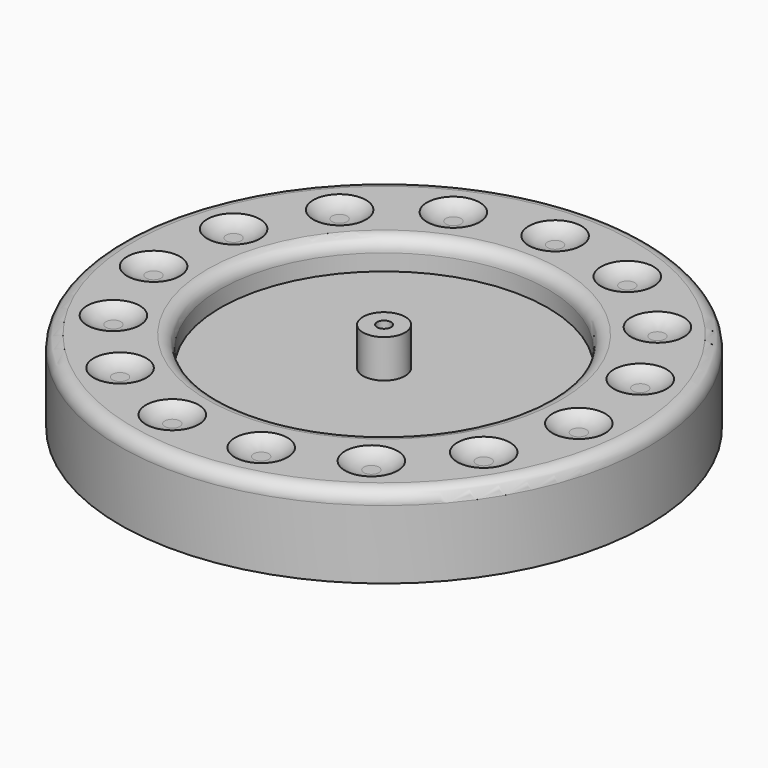
from build123d import *

# Parameters (mm, degrees)
F0_R      = 50
F1_DEPTH  = 15.5
F2_R      = 31
F3_DEPTH  = 7.1
F4_R      = 11.125
F5_DEPTH  = 9
F6_R      = 2.5
F7_R      = 5
F8_DEPTH  = 1.5
F10_R     = 31.0625
F11_DEPTH = 1.5
F12_R     = 4
F13_DEPTH = 7.25
F15_D     = 2.65
F15_DEPTH = 10
F15_TIP   = 0.7961403202


# Not quite as in the source:
# - a fillet or chamfer that OpenCascade refuses, or shapes differently, is made with other operations: its cross-section is extruded or revolved along the edge and cut away or added


with BuildPart() as f1:
    # F0 (on Top) → F1 (new body)
    with BuildSketch(Plane.XY):
        Circle(F0_R)
    extrude(amount=F1_DEPTH)

    # F2 (on face) → F3 (cut)
    with BuildSketch(Plane.XY.offset(15.5)):
        Circle(F2_R)
    extrude(amount=-F3_DEPTH, mode=Mode.SUBTRACT)

    # F4 (on face) → F5 (cut)
    with BuildSketch(Plane.XY.offset(8.4)):
        Circle(F4_R)
    extrude(amount=-F5_DEPTH, mode=Mode.SUBTRACT)

    # F6
    f6_edges = [f1.edges().sort_by_distance(p)[0] for p in [
        (-50, 0, 15.5),
        (-31, 0, 15.5),
    ]]
    fillet(f6_edges, radius=F6_R)

    # F7 (on face) → F8 (cut)
    with BuildSketch(Plane.XY.offset(15.5)):
        with Locations((0, 40.5)):
            Circle(F7_R)
        with Locations((-16.4728340446, 36.9985910345)):
            Circle(F7_R)
        with Locations((-30.0973654318, 27.0997895575)):
            Circle(F7_R)
        with Locations((-38.51778891, 12.5151882722)):
            Circle(F7_R)
        with Locations((-40.2781367624, -4.2334027623)):
            Circle(F7_R)
        with Locations((-35.0740288533, -20.25)):
            Circle(F7_R)
        with Locations((-23.8053027178, -32.7651882722)):
            Circle(F7_R)
        with Locations((-8.4204234781, -39.6149778297)):
            Circle(F7_R)
        with Locations((8.4204234781, -39.6149778297)):
            Circle(F7_R)
        with Locations((23.8053027178, -32.7651882722)):
            Circle(F7_R)
        with Locations((35.0740288533, -20.25)):
            Circle(F7_R)
        with Locations((40.2781367624, -4.2334027623)):
            Circle(F7_R)
        with Locations((38.51778891, 12.5151882722)):
            Circle(F7_R)
        with Locations((30.0973654318, 27.0997895575)):
            Circle(F7_R)
        with Locations((16.4728340446, 36.9985910345)):
            Circle(F7_R)
    extrude(amount=-F8_DEPTH, mode=Mode.SUBTRACT)

    # F9: fillet of radius 5 on 15 edges, made by hand

    # F9_s1 → F9_t2 (revolve)
    with BuildSketch(Plane.XZ.offset(-40.5)):
        with BuildLine():
            ThreePointArc((5, 15.5), (3.3657774588, 14.3902277714), (1.4292857857, 14))
            Line((1.4292857857, 14), (5, 14))
            Line((5, 14), (5, 15.5))
        make_face()
    revolve(axis=Axis((0, 40.5, 14), (0, 0, 1)))

    # F9_s3 → F9_t4 (revolve)
    with BuildSketch(Plane.XZ.offset(-36.9985910345)):
        with BuildLine():
            ThreePointArc((-11.4728340446, 15.5), (-13.1070565857, 14.3902277714), (-15.0435482588, 14))
            Line((-15.0435482588, 14), (-11.4728340446, 14))
            Line((-11.4728340446, 14), (-11.4728340446, 15.5))
        make_face()
    revolve(axis=Axis((-16.4728340446, 36.9985910345, 14), (0, 0, 1)))

    # F9_s5 → F9_t6 (revolve)
    with BuildSketch(Plane.XZ.offset(-27.0997895575)):
        with BuildLine():
            ThreePointArc((-25.0973654318, 15.5), (-26.731587973, 14.3902277714), (-28.6680796461, 14))
            Line((-28.6680796461, 14), (-25.0973654318, 14))
            Line((-25.0973654318, 14), (-25.0973654318, 15.5))
        make_face()
    revolve(axis=Axis((-30.0973654318, 27.0997895575, 14), (0, 0, 1)))

    # F9_s7 → F9_t8 (revolve)
    with BuildSketch(Plane.XZ.offset(-12.5151882722)):
        with BuildLine():
            ThreePointArc((-33.51778891, 15.5), (-35.1520114511, 14.3902277714), (-37.0885031242, 14))
            Line((-37.0885031242, 14), (-33.51778891, 14))
            Line((-33.51778891, 14), (-33.51778891, 15.5))
        make_face()
    revolve(axis=Axis((-38.51778891, 12.5151882722, 14), (0, 0, 1)))

    # F9_s9 → F9_t10 (revolve)
    with BuildSketch(Plane.XZ.offset(4.2334027623)):
        with BuildLine():
            ThreePointArc((-35.2781367624, 15.5), (-36.9123593036, 14.3902277714), (-38.8488509767, 14))
            Line((-38.8488509767, 14), (-35.2781367624, 14))
            Line((-35.2781367624, 14), (-35.2781367624, 15.5))
        make_face()
    revolve(axis=Axis((-40.2781367624, -4.2334027623, 14), (0, 0, 1)))

    # F9_s11 → F9_t12 (revolve)
    with BuildSketch(Plane.XZ.offset(20.25)):
        with BuildLine():
            ThreePointArc((-30.0740288533, 15.5), (-31.7082513944, 14.3902277714), (-33.6447430675, 14))
            Line((-33.6447430675, 14), (-30.0740288533, 14))
            Line((-30.0740288533, 14), (-30.0740288533, 15.5))
        make_face()
    revolve(axis=Axis((-35.0740288533, -20.25, 14), (0, 0, 1)))

    # F9_s13 → F9_t14 (revolve)
    with BuildSketch(Plane.XZ.offset(32.7651882722)):
        with BuildLine():
            ThreePointArc((-18.8053027178, 15.5), (-20.439525259, 14.3902277714), (-22.3760169321, 14))
            Line((-22.3760169321, 14), (-18.8053027178, 14))
            Line((-18.8053027178, 14), (-18.8053027178, 15.5))
        make_face()
    revolve(axis=Axis((-23.8053027178, -32.7651882722, 14), (0, 0, 1)))

    # F9_s15 → F9_t16 (revolve)
    with BuildSketch(Plane.XZ.offset(39.6149778297)):
        with BuildLine():
            ThreePointArc((-3.4204234781, 15.5), (-5.0546460193, 14.3902277714), (-6.9911376924, 14))
            Line((-6.9911376924, 14), (-3.4204234781, 14))
            Line((-3.4204234781, 14), (-3.4204234781, 15.5))
        make_face()
    revolve(axis=Axis((-8.4204234781, -39.6149778297, 14), (0, 0, 1)))

    # F9_s17 → F9_t18 (revolve)
    with BuildSketch(Plane.XZ.offset(39.6149778297)):
        with BuildLine():
            ThreePointArc((13.4204234781, 15.5), (11.786200937, 14.3902277714), (9.8497092638, 14))
            Line((9.8497092638, 14), (13.4204234781, 14))
            Line((13.4204234781, 14), (13.4204234781, 15.5))
        make_face()
    revolve(axis=Axis((8.4204234781, -39.6149778297, 14), (0, 0, 1)))

    # F9_s19 → F9_t20 (revolve)
    with BuildSketch(Plane.XZ.offset(32.7651882722)):
        with BuildLine():
            ThreePointArc((28.8053027178, 15.5), (27.1710801767, 14.3902277714), (25.2345885036, 14))
            Line((25.2345885036, 14), (28.8053027178, 14))
            Line((28.8053027178, 14), (28.8053027178, 15.5))
        make_face()
    revolve(axis=Axis((23.8053027178, -32.7651882722, 14), (0, 0, 1)))

    # F9_s21 → F9_t22 (revolve)
    with BuildSketch(Plane.XZ.offset(20.25)):
        with BuildLine():
            ThreePointArc((40.0740288533, 15.5), (38.4398063121, 14.3902277714), (36.503314639, 14))
            Line((36.503314639, 14), (40.0740288533, 14))
            Line((40.0740288533, 14), (40.0740288533, 15.5))
        make_face()
    revolve(axis=Axis((35.0740288533, -20.25, 14), (0, 0, 1)))

    # F9_s23 → F9_t24 (revolve)
    with BuildSketch(Plane.XZ.offset(4.2334027623)):
        with BuildLine():
            ThreePointArc((45.2781367624, 15.5), (43.6439142212, 14.3902277714), (41.7074225481, 14))
            Line((41.7074225481, 14), (45.2781367624, 14))
            Line((45.2781367624, 14), (45.2781367624, 15.5))
        make_face()
    revolve(axis=Axis((40.2781367624, -4.2334027623, 14), (0, 0, 1)))

    # F9_s25 → F9_t26 (revolve)
    with BuildSketch(Plane.XZ.offset(-12.5151882722)):
        with BuildLine():
            ThreePointArc((43.51778891, 15.5), (41.8835663688, 14.3902277714), (39.9470746957, 14))
            Line((39.9470746957, 14), (43.51778891, 14))
            Line((43.51778891, 14), (43.51778891, 15.5))
        make_face()
    revolve(axis=Axis((38.51778891, 12.5151882722, 14), (0, 0, 1)))

    # F9_s27 → F9_t28 (revolve)
    with BuildSketch(Plane.XZ.offset(-27.0997895575)):
        with BuildLine():
            ThreePointArc((35.0973654318, 15.5), (33.4631428907, 14.3902277714), (31.5266512176, 14))
            Line((31.5266512176, 14), (35.0973654318, 14))
            Line((35.0973654318, 14), (35.0973654318, 15.5))
        make_face()
    revolve(axis=Axis((30.0973654318, 27.0997895575, 14), (0, 0, 1)))

    # F9_s29 → F9_t30 (revolve)
    with BuildSketch(Plane.XZ.offset(-36.9985910345)):
        with BuildLine():
            ThreePointArc((21.4728340446, 15.5), (19.8386115034, 14.3902277714), (17.9021198303, 14))
            Line((17.9021198303, 14), (21.4728340446, 14))
            Line((21.4728340446, 14), (21.4728340446, 15.5))
        make_face()
    revolve(axis=Axis((16.4728340446, 36.9985910345, 14), (0, 0, 1)))

    # F10 (on face) → F11 (join)
    with BuildSketch(Plane.XY.offset(8.4)):
        Circle(F10_R)
    extrude(amount=F11_DEPTH)

    # F12 (on face) → F13 (join)
    with BuildSketch(Plane.XY.offset(9.9)):
        Circle(F12_R)
    extrude(amount=F13_DEPTH)

    # F15
    with Locations(Plane.XY.offset(17.15)):
        with Locations((0, 0)):
            Hole(F15_D / 2, depth=F15_DEPTH)
            with Locations((0, 0, -(F15_DEPTH + F15_TIP / 2))):  # 118° drill point
                Cone(0, F15_D / 2, F15_TIP, mode=Mode.SUBTRACT)


solid = f1.part
